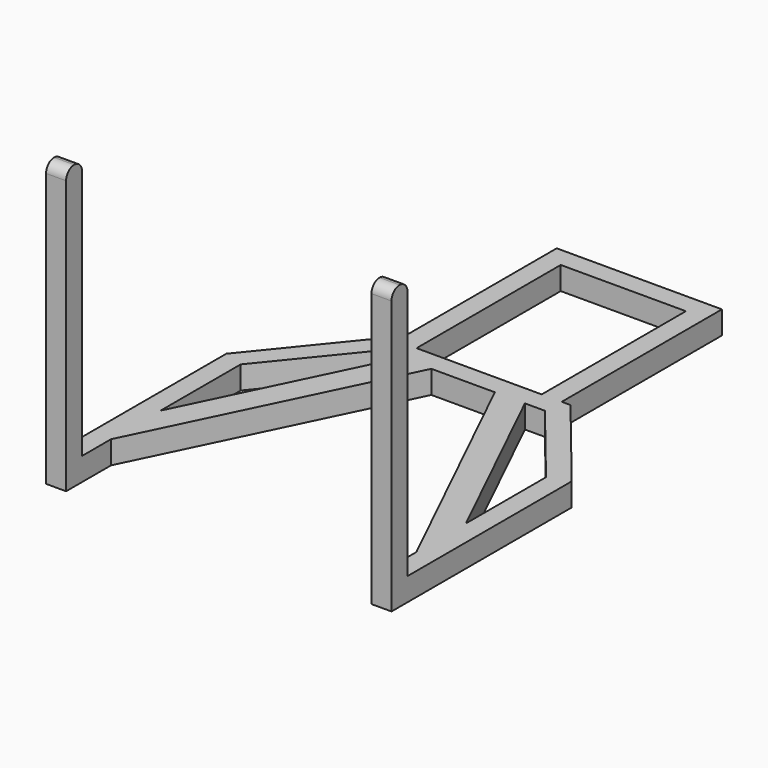
from build123d import *

# Parameters (mm, degrees)
F1_DEPTH = 4.6
F2_W     = 4
F2_H     = 4
F3_DEPTH = 52
F4_R     = 1.99999


# Not quite as in the source:
# - a fillet or chamfer is up to 0.001 mm smaller than in the source, because OpenCascade refuses the exact size


with BuildPart() as f1:
    # F0 (on Top) → F1 (new body)
    with BuildSketch(Plane.XY):
        Polygon((16.5, 0), (-16.5, 0), (-16.5, -40), (-12.5, -40), (-12.5, -4), (12.5, -4), (12.5, -40), (16.5, -40), align=None)
        Polygon((-12.5, -40), (-16.5, -40), (-18.25, -40), (-34.5, -60), (-34.5, -105), (-30.5, -105), (-30.5, -93.7917722906), (-30.5, -81.420162501), (-30.5, -61.420162501), (-16.346117968, -44), (-12.346117968, -44), (-6.344200027, -44), (6.344200027, -44), (12.346117968, -44), (16.346117968, -44), (30.5, -61.420162501), (30.5, -81.420162501), (30.5, -93.7917722906), (30.5, -105), (34.5, -105), (34.5, -60), (18.25, -40), (16.5, -40), (12.5, -40), align=None)
        Polygon((-30.5, -81.420162501), (-30.5, -93.7917722906), (-6.344200027, -44), (-12.346117968, -44), align=None)
        Polygon((6.344200027, -44), (30.5, -93.7917722906), (30.5, -81.420162501), (12.346117968, -44), align=None)
    extrude(amount=F1_DEPTH)

    # F2 (on face) → F3 (join)
    with BuildSketch(Plane.XY.offset(4.6)):
        with Locations((-32.5, -103)):
            Rectangle(F2_W, F2_H)
        with Locations((32.5, -103)):
            Rectangle(F2_W, F2_H)
    extrude(amount=F3_DEPTH)

    # F4 (radius 2 in the source; OpenCascade refuses exactly that, so slightly less here)
    f4_edges = [f1.edges().sort_by_distance(p)[0] for p in [
        (-32.5, -105, 56.6),
        (-32.5, -101, 56.6),
        (32.5, -105, 56.6),
        (32.5, -101, 56.6),
    ]]
    fillet(f4_edges, radius=F4_R)


solid = f1.part
